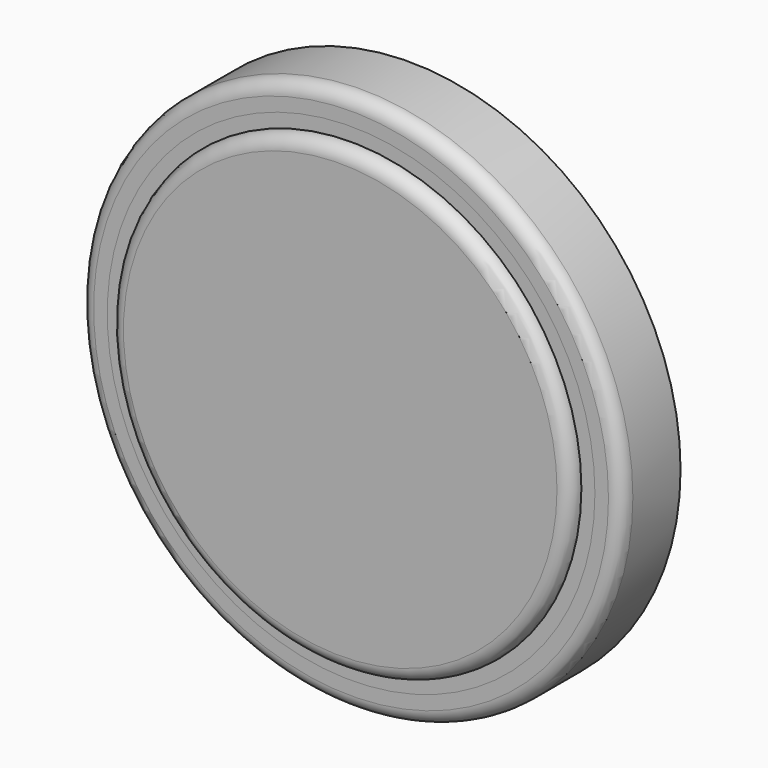
from build123d import *

# Parameters (mm, degrees)
F0_R     = 8.5
F1_DEPTH = 3.2
F0_R_2   = 9
F2_DEPTH = 2.2
F0_R_3   = 10
F3_DEPTH = 2.7
F4_R     = 0.5
F5_R     = 0.5
F7_DEPTH = 0.5
F9_DEPTH = 0.5


# Not quite as in the source:
# - a feature names something its author has since deleted; it is built from what else it names


with BuildPart() as f1:
    # F0 (on Front) → F1 (new body)
    with BuildSketch(Plane.XZ):
        Circle(F0_R)
    extrude(amount=F1_DEPTH)

    # F5
    f5_edges = [f1.edges().sort_by_distance(p)[0] for p in [
        (-8.5, -3.2, 0),
    ]]
    fillet(f5_edges, radius=F5_R)



with BuildPart() as f2:
    # F0 (on Front) → F2 (new body)
    with BuildSketch(Plane.XZ):
        Circle(F0_R_2)
        Circle(F0_R, mode=Mode.SUBTRACT)
    extrude(amount=F2_DEPTH)


with BuildPart() as f3:
    # F0 (on Front) → F3 (new body)
    with BuildSketch(Plane.XZ):
        Circle(F0_R_3)
        Circle(F0_R_2, mode=Mode.SUBTRACT)
    extrude(amount=F3_DEPTH)

    # F4
    f4_edges = [f3.edges().sort_by_distance(p)[0] for p in [
        (-10, -2.7, 0),
    ]]
    fillet(f4_edges, radius=F4_R)


with BuildPart() as f2_1:
    # F6: moved
    add(f2.part.moved(Location((0, -0.5, 0))))


with BuildPart() as f7:
    # F7 (new): a face of the model
    f7_faces = [f3.part.faces().sort_by_distance(p)[0] for p in [
        (-9.2312994231, -2.7, 0),
    ]]
    extrude(f7_faces, amount=F7_DEPTH)


with BuildPart() as f1_1:
    add(f1.part)

    add(f3.part)  # F9 merges F3
    # F0 (on Front) → F9 (join)
    with BuildSketch(Plane.XZ):
        Circle(F0_R_2)
        Circle(F0_R, mode=Mode.SUBTRACT)
    extrude(amount=F9_DEPTH)


solid = Compound([f2_1.part, f1_1.part])
